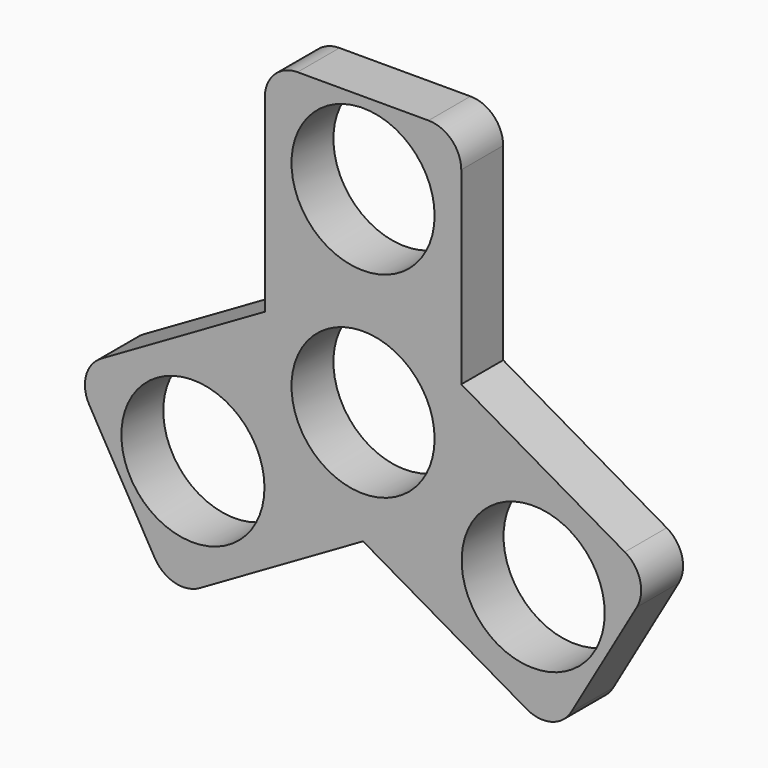
from build123d import *

# Parameters (mm, degrees)
F0_R     = 10.925
F1_DEPTH = 8


with BuildPart() as f1:
    # F0 (on Front) → F1 (new body)
    with BuildSketch(Plane.XZ):
        with BuildLine():
            ThreePointArc((-145.8578413725, 37.5421847403), (-147.3223074666, 41.0777186462), (-150.8578413725, 42.5421847403))
            Line((-150.8578413725, 42.5421847403), (-170.8578413725, 42.5421847403))
            ThreePointArc((-170.8578413725, 42.5421847403), (-174.3933752784, 41.0777186462), (-175.8578413725, 37.5421847403))
            Line((-175.8578413725, 37.5421847403), (-175.8578413725, 8.7024387781))
            Line((-175.8578413725, 8.7024387781), (-167.5084764671, 13.5229468538))
            Line((-167.5084764671, 13.5229468538), (-164.1831589198, 19.2825657971))
            Line((-164.1831589198, 19.2825657971), (-160.8578413725, 17.362692816))
            Line((-160.8578413725, 17.362692816), (-157.5325238252, 19.2825657971))
            Line((-157.5325238252, 19.2825657971), (-154.2072062779, 13.5229468538))
            Line((-154.2072062779, 13.5229468538), (-145.8578413725, 8.7024387781))
            Line((-145.8578413725, 8.7024387781), (-145.8578413725, 37.5421847403))
        make_face()
        with Locations((-160.8578413725, 30.0421847403)):
            Circle(F0_R, mode=Mode.SUBTRACT)
        with BuildLine():
            Line((-120.8818887306, -5.7174342029), (-145.8578413725, 8.7024387781))
            Line((-145.8578413725, 8.7024387781), (-145.8578413725, -0.9385773732))
            Line((-145.8578413725, -0.9385773732), (-142.5325238252, -6.6981963165))
            Line((-142.5325238252, -6.6981963165), (-145.8578413725, -8.6180692975))
            Line((-145.8578413725, -8.6180692975), (-145.8578413725, -12.4578152597))
            Line((-145.8578413725, -12.4578152597), (-152.5084764671, -12.4578152597))
            Line((-152.5084764671, -12.4578152597), (-160.8578413725, -17.2783233354))
            Line((-160.8578413725, -17.2783233354), (-135.8818887306, -31.6981963165))
            ThreePointArc((-135.8818887306, -31.6981963165), (-132.0877935051, -32.197698429), (-129.0517617117, -29.8680692975))
            Line((-129.0517617117, -29.8680692975), (-119.0517617117, -12.5475612219))
            ThreePointArc((-119.0517617117, -12.5475612219), (-118.5522595991, -8.7534659963), (-120.8818887306, -5.7174342029))
        make_face()
        with Locations((-134.877079259, -14.9578152597)):
            Circle(F0_R, mode=Mode.SUBTRACT)
        Polygon((-145.8578413725, -0.9385773732), (-145.8578413725, 8.7024387781), (-154.2072062779, 13.5229468538), align=None)
        Polygon((-167.5084764671, 13.5229468538), (-175.8578413725, 8.7024387781), (-175.8578413725, -0.9385773732), align=None)
        with BuildLine():
            Line((-175.8578413725, -0.9385773732), (-175.8578413725, 8.7024387781))
            Line((-175.8578413725, 8.7024387781), (-200.8337940144, -5.7174342029))
            ThreePointArc((-200.8337940144, -5.7174342029), (-203.1634231459, -8.7534659963), (-202.6639210333, -12.5475612219))
            Line((-202.6639210333, -12.5475612219), (-192.6639210333, -29.8680692975))
            ThreePointArc((-192.6639210333, -29.8680692975), (-189.6278892399, -32.197698429), (-185.8337940144, -31.6981963165))
            Line((-185.8337940144, -31.6981963165), (-160.8578413725, -17.2783233354))
            Line((-160.8578413725, -17.2783233354), (-169.2072062779, -12.4578152597))
            Line((-169.2072062779, -12.4578152597), (-175.8578413725, -12.4578152597))
            Line((-175.8578413725, -12.4578152597), (-175.8578413725, -8.6180692975))
            Line((-175.8578413725, -8.6180692975), (-179.1831589198, -6.6981963165))
            Line((-179.1831589198, -6.6981963165), (-175.8578413725, -0.9385773732))
        make_face()
        with Locations((-186.838603486, -14.9578152597)):
            Circle(F0_R, mode=Mode.SUBTRACT)
        Polygon((-160.8578413725, -17.2783233354), (-152.5084764671, -12.4578152597), (-169.2072062779, -12.4578152597), align=None)
        Polygon((-145.8578413725, -8.6180692975), (-145.8578413725, -0.9385773732), (-154.2072062779, 13.5229468538), (-160.8578413725, 17.362692816), (-167.5084764671, 13.5229468538), (-175.8578413725, -0.9385773732), (-175.8578413725, -8.6180692975), (-169.2072062779, -12.4578152597), (-152.5084764671, -12.4578152597), align=None)
        with Locations((-160.8578413725, 0.0421847403)):
            Circle(F0_R, mode=Mode.SUBTRACT)
        Polygon((-142.5325238252, -6.6981963165), (-145.8578413725, -0.9385773732), (-145.8578413725, -8.6180692975), align=None)
        Polygon((-145.8578413725, -12.4578152597), (-145.8578413725, -8.6180692975), (-152.5084764671, -12.4578152597), align=None)
        Polygon((-169.2072062779, -12.4578152597), (-175.8578413725, -8.6180692975), (-175.8578413725, -12.4578152597), align=None)
        Polygon((-175.8578413725, -8.6180692975), (-175.8578413725, -0.9385773732), (-179.1831589198, -6.6981963165), align=None)
        Polygon((-164.1831589198, 19.2825657971), (-167.5084764671, 13.5229468538), (-160.8578413725, 17.362692816), align=None)
        Polygon((-160.8578413725, 17.362692816), (-154.2072062779, 13.5229468538), (-157.5325238252, 19.2825657971), align=None)
    extrude(amount=F1_DEPTH)


solid = f1.part
